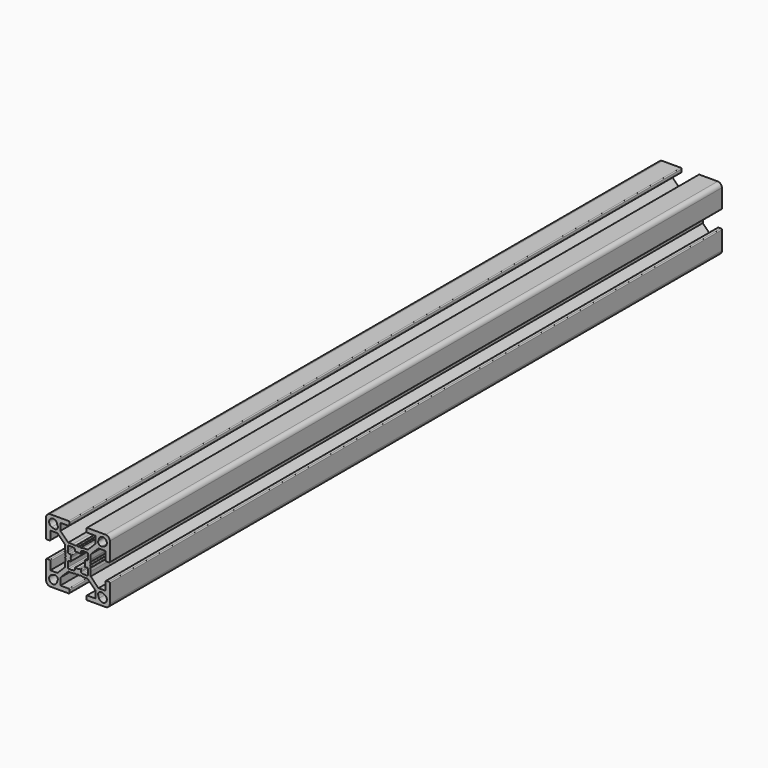
from build123d import *

# Parameters (mm, degrees)
F1_DEPTH = 360


# Not quite as in the source:
# - ends of sketch curves that miss each other by under 0.0002 mm in the source are joined


with BuildPart() as f1:
    # F0 (on Front) → F1 (new body)
    with BuildSketch(Plane.XZ):
        with BuildLine():
            ThreePointArc((21.683673, 22.959406), (21.8008302875, 23.2422487125), (22.083673, 23.359406))
            Line((22.083673, 23.359406), (23.829607, 23.359406))
            ThreePointArc((23.829607, 23.359406), (23.8679454853, 23.3575644616), (23.9059309617, 23.3520568027))
            Line((23.9059309617, 23.3520568027), (24.659993, 23.205482))
            ThreePointArc((24.659993, 23.205482), (24.8923196389, 23.067262524), (24.98367, 22.812831))
            Line((24.98367, 22.812831), (24.98367, 22.196712))
            ThreePointArc((24.98367, 22.196712), (25.1452540389, 21.8755300741), (25.4994591475, 21.8138375123))
            ThreePointArc((25.4994591475, 21.8138375123), (25.9862111121, 21.9228171635), (26.48367, 21.959406))
            Line((26.48367, 21.959406), (26.48367, 24.259406))
            Line((26.48367, 24.259406), (26.080079, 24.492418))
            ThreePointArc((26.080079, 24.492418), (25.830079, 24.559406), (25.5800791291, 24.4924187764))
            Line((25.5800791291, 24.4924187764), (25.264783, 24.310382))
            Line((25.264783, 24.310382), (23.98367, 24.559406))
            Line((23.98367, 24.559406), (21.897875, 24.559406))
            Line((21.897875, 24.559406), (18.23367, 28.223612))
            Line((18.23367, 28.223612), (18.23367, 31.559402))
            Line((18.23367, 31.559402), (22.083673, 31.559402))
            ThreePointArc((22.083673, 31.559402), (22.3665157125, 31.6765592875), (22.483673, 31.959402))
            Line((22.483673, 31.959402), (22.483673, 33.159402))
            ThreePointArc((22.483673, 33.159402), (22.3665157125, 33.4422447125), (22.083673, 33.559402))
            Line((22.083673, 33.559402), (13.483674, 33.559402))
            ThreePointArc((13.483674, 33.559402), (12.0694604376, 32.9736155624), (11.483674, 31.559402))
            Line((11.483674, 31.559402), (11.483674, 22.959403))
            ThreePointArc((11.483674, 22.959403), (11.6008312875, 22.6765602875), (11.883674, 22.559403))
            Line((11.883674, 22.559403), (13.083674, 22.559403))
            ThreePointArc((13.083674, 22.559403), (13.3665167125, 22.6765602875), (13.483674, 22.959403))
            Line((13.483674, 22.959403), (13.483674, 26.809406))
            Line((13.483674, 26.809406), (16.819447, 26.809406))
            Line((16.819447, 26.809406), (20.48367, 23.145184))
            Line((20.48367, 23.145184), (20.48367, 21.059406))
            Line((20.48367, 21.059406), (20.732693, 19.778291))
            Line((20.732693, 19.778291), (20.550657, 19.462994))
            ThreePointArc((20.550657, 19.462994), (20.48367, 19.212994), (20.5506572236, 18.9629941291))
            Line((20.5506572236, 18.9629941291), (20.78367, 18.559405))
            Line((20.78367, 18.559405), (23.08367, 18.559406))
            ThreePointArc((23.08367, 18.559406), (23.1202587453, 19.0568642713), (23.2292374892, 19.543615852))
            ThreePointArc((23.2292374892, 19.543615852), (23.1675451248, 19.897821693), (22.846363, 20.059406))
            Line((22.846363, 20.059406), (22.230245, 20.059406))
            ThreePointArc((22.230245, 20.059406), (21.9758138548, 20.1507560489), (21.8375941973, 20.3830820383))
            Line((21.8375941973, 20.3830820383), (21.691022, 21.137129))
            ThreePointArc((21.691022, 21.137129), (21.6855145384, 21.1751145147), (21.683673, 21.213453))
            Line((21.683673, 21.213453), (21.683673, 22.959406))
        make_face()
        with BuildLine():
            ThreePointArc((14.1338310917, 28.473990252), (13.440167448, 31.6029092165), (16.5690860694, 30.9092440253))
            Line((16.5690860694, 30.9092440253), (16.935818, 29.901655))
            ThreePointArc((16.935818, 29.901655), (16.610197705, 28.4328777176), (15.1414197615, 28.1072573447))
            Line((15.1414197615, 28.1072573447), (14.1338310917, 28.473990252))
        make_face(mode=Mode.SUBTRACT)
        with BuildLine():
            Line((26.48367, 24.259406), (26.48367, 21.959406))
            ThreePointArc((26.48367, 21.959406), (26.9811284145, 21.9228172335), (27.4678801291, 21.813838427))
            ThreePointArc((27.4678801291, 21.813838427), (27.8220855768, 21.8755297889), (27.98367, 22.196712))
            Line((27.98367, 22.196712), (27.98367, 22.812831))
            ThreePointArc((27.98367, 22.812831), (28.0750200489, 23.0672621452), (28.3073460383, 23.2054818027))
            Line((28.3073460383, 23.2054818027), (29.061393, 23.352053))
            ThreePointArc((29.061393, 23.352053), (29.0993785147, 23.3575614616), (29.137717, 23.359403))
            Line((29.137717, 23.359403), (30.88367, 23.359403))
            ThreePointArc((30.88367, 23.359403), (31.1665127125, 23.2422457125), (31.28367, 22.959403))
            Line((31.28367, 22.959403), (31.28367, 21.213468))
            ThreePointArc((31.28367, 21.213468), (31.2818285086, 21.1751300032), (31.27632099, 21.1371450019))
            Line((31.27632099, 21.1371450019), (31.129746, 20.383082))
            ThreePointArc((31.129746, 20.383082), (30.9915261452, 20.1507560489), (30.737095, 20.059406))
            Line((30.737095, 20.059406), (30.120976, 20.059406))
            ThreePointArc((30.120976, 20.059406), (29.7997937889, 19.8978215768), (29.7381017894, 19.5436159363))
            ThreePointArc((29.7381017894, 19.5436159363), (29.8470812335, 19.0568644145), (29.88367, 18.559406))
            Line((29.88367, 18.559406), (32.18367, 18.559406))
            Line((32.18367, 18.559406), (32.416682, 18.962996))
            ThreePointArc((32.416682, 18.962996), (32.48367, 19.212996), (32.4166825264, 19.4629963039))
            Line((32.4166825264, 19.4629963039), (32.234646, 19.778292))
            Line((32.234646, 19.778292), (32.48367, 21.059406))
            Line((32.48367, 21.059406), (32.48367, 23.1452))
            Line((32.48367, 23.1452), (36.147876, 26.809406))
            Line((36.147876, 26.809406), (39.483666, 26.809406))
            Line((39.483666, 26.809406), (39.483666, 22.959403))
            ThreePointArc((39.483666, 22.959403), (39.6008232875, 22.6765602875), (39.883666, 22.559403))
            Line((39.883666, 22.559403), (41.083666, 22.559403))
            ThreePointArc((41.083666, 22.559403), (41.3665087125, 22.6765602875), (41.483666, 22.959403))
            Line((41.483666, 22.959403), (41.483666, 31.559402))
            ThreePointArc((41.483666, 31.559402), (40.8978795624, 32.9736155624), (39.483666, 33.559402))
            Line((39.483666, 33.559402), (30.883667, 33.559402))
            ThreePointArc((30.883667, 33.559402), (30.6008242875, 33.4422447125), (30.483667, 33.159402))
            Line((30.483667, 33.159402), (30.483667, 31.959402))
            ThreePointArc((30.483667, 31.959402), (30.6008242875, 31.6765592875), (30.883667, 31.559402))
            Line((30.883667, 31.559402), (34.73367, 31.559402))
            Line((34.73367, 31.559402), (34.73367, 28.223628))
            Line((34.73367, 28.223628), (31.069448, 24.559406))
            Line((31.069448, 24.559406), (28.98367, 24.559406))
            Line((28.98367, 24.559406), (27.702555, 24.310382))
            Line((27.702555, 24.310382), (27.387259, 24.492418))
            ThreePointArc((27.387259, 24.492418), (27.137259, 24.559406), (26.8872591291, 24.4924187764))
            Line((26.8872591291, 24.4924187764), (26.48367, 24.259406))
        make_face()
        with BuildLine():
            ThreePointArc((36.3982539306, 30.9092440253), (39.5271728843, 31.6029088843), (38.8335080253, 28.4739899306))
            Line((38.8335080253, 28.4739899306), (37.825919, 28.107257))
            ThreePointArc((37.825919, 28.107257), (36.3571411741, 28.4328778386), (36.0315216661, 29.9016561215))
            Line((36.0315216661, 29.9016561215), (36.3982539306, 30.9092440253))
        make_face(mode=Mode.SUBTRACT)
        with BuildLine():
            ThreePointArc((23.2292377663, 17.5751952317), (23.1202588153, 18.0619472552), (23.08367, 18.559406))
            Line((23.08367, 18.559406), (20.78367, 18.559406))
            Line((20.78367, 18.559406), (20.550657, 18.155815))
            ThreePointArc((20.550657, 18.155815), (20.48367, 17.905815), (20.5506572236, 17.6558151291))
            Line((20.5506572236, 17.6558151291), (20.732693, 17.340519))
            Line((20.732693, 17.340519), (20.48367, 16.059406))
            Line((20.48367, 16.059406), (20.48367, 13.973611))
            Line((20.48367, 13.973611), (16.819464, 10.309406))
            Line((16.819464, 10.309406), (13.483674, 10.309406))
            Line((13.483674, 10.309406), (13.483674, 14.159409))
            ThreePointArc((13.483674, 14.159409), (13.3665167125, 14.4422517125), (13.083674, 14.559409))
            Line((13.083674, 14.559409), (11.883674, 14.559409))
            ThreePointArc((11.883674, 14.559409), (11.6008312875, 14.4422517125), (11.483674, 14.159409))
            Line((11.483674, 14.159409), (11.483674, 5.55941))
            ThreePointArc((11.483674, 5.55941), (12.0694604376, 4.1451964376), (13.483674, 3.55941))
            Line((13.483674, 3.55941), (22.083673, 3.55941))
            ThreePointArc((22.083673, 3.55941), (22.3665157125, 3.6765672875), (22.483673, 3.95941))
            Line((22.483673, 3.95941), (22.483673, 5.15941))
            ThreePointArc((22.483673, 5.15941), (22.3665157125, 5.4422527125), (22.083673, 5.55941))
            Line((22.083673, 5.55941), (18.23367, 5.55941))
            Line((18.23367, 5.55941), (18.23367, 8.895183))
            Line((18.23367, 8.895183), (21.897891, 12.559406))
            Line((21.897891, 12.559406), (23.98367, 12.559406))
            Line((23.98367, 12.559406), (25.264785, 12.808429))
            Line((25.264785, 12.808429), (25.580081, 12.626393))
            ThreePointArc((25.580081, 12.626393), (25.830081, 12.559406), (26.0800808709, 12.6263932236))
            Line((26.0800808709, 12.6263932236), (26.483671, 12.859406))
            Line((26.483671, 12.859406), (26.48367, 15.159406))
            ThreePointArc((26.48367, 15.159406), (25.9862111121, 15.1959948365), (25.4994589547, 15.3049738501))
            ThreePointArc((25.4994589547, 15.3049738501), (25.1452540389, 15.2432809259), (24.98367, 14.922099))
            Line((24.98367, 14.922099), (24.98367, 14.305981))
            ThreePointArc((24.98367, 14.305981), (24.8923196389, 14.051549476), (24.6599929981, 13.91333001))
            Line((24.6599929981, 13.91333001), (23.905946, 13.766758))
            ThreePointArc((23.905946, 13.766758), (23.8679609968, 13.7612504914), (23.829623, 13.759409))
            Line((23.829623, 13.759409), (22.08367, 13.759409))
            ThreePointArc((22.08367, 13.759409), (21.8008272875, 13.8765662875), (21.68367, 14.159409))
            Line((21.68367, 14.159409), (21.68367, 15.905343))
            ThreePointArc((21.68367, 15.905343), (21.6855115384, 15.9436814853), (21.6910191973, 15.9816669617))
            Line((21.6910191973, 15.9816669617), (21.837594, 16.735729))
            ThreePointArc((21.837594, 16.735729), (21.975813476, 16.9680556389), (22.230245, 17.059406))
            Line((22.230245, 17.059406), (22.846363, 17.059406))
            ThreePointArc((22.846363, 17.059406), (23.1675448396, 17.2209899227), (23.2292377663, 17.5751952317))
        make_face()
        with BuildLine():
            ThreePointArc((16.5690860694, 6.2095679747), (13.440167448, 5.5159027835), (14.1338310917, 8.644821748))
            Line((14.1338310917, 8.644821748), (15.14142, 9.011554))
            ThreePointArc((15.14142, 9.011554), (16.6101974937, 8.6859334937), (16.9358177723, 7.2171560829))
            Line((16.9358177723, 7.2171560829), (16.5690860694, 6.2095679747))
        make_face(mode=Mode.SUBTRACT)
        with BuildLine():
            ThreePointArc((27.4678801291, 15.304973573), (26.9811284145, 15.1959947665), (26.48367, 15.159406))
            Line((26.48367, 15.159406), (26.48367, 12.859406))
            Line((26.48367, 12.859406), (26.887261, 12.626393))
            ThreePointArc((26.887261, 12.626393), (27.137261, 12.559406), (27.3872608709, 12.6263932236))
            Line((27.3872608709, 12.6263932236), (27.702556, 12.808429))
            Line((27.702556, 12.808429), (28.98367, 12.559406))
            Line((28.98367, 12.559406), (31.069464, 12.559406))
            Line((31.069464, 12.559406), (34.73367, 8.8952))
            Line((34.73367, 8.8952), (34.73367, 5.55941))
            Line((34.73367, 5.55941), (30.883667, 5.55941))
            ThreePointArc((30.883667, 5.55941), (30.6008242875, 5.4422527125), (30.483667, 5.15941))
            Line((30.483667, 5.15941), (30.483667, 3.95941))
            ThreePointArc((30.483667, 3.95941), (30.6008242875, 3.6765672875), (30.883667, 3.55941))
            Line((30.883667, 3.55941), (39.483666, 3.55941))
            ThreePointArc((39.483666, 3.55941), (40.8978795624, 4.1451964376), (41.483666, 5.55941))
            Line((41.483666, 5.55941), (41.483666, 14.159409))
            ThreePointArc((41.483666, 14.159409), (41.3665087125, 14.4422517125), (41.083666, 14.559409))
            Line((41.083666, 14.559409), (39.883666, 14.559409))
            ThreePointArc((39.883666, 14.559409), (39.6008232875, 14.4422517125), (39.483666, 14.159409))
            Line((39.483666, 14.159409), (39.483666, 10.309406))
            Line((39.483666, 10.309406), (36.147892, 10.309406))
            Line((36.147892, 10.309406), (32.48367, 13.973627))
            Line((32.48367, 13.973627), (32.48367, 16.059406))
            Line((32.48367, 16.059406), (32.234646, 17.340521))
            Line((32.234646, 17.340521), (32.416682, 17.655817))
            ThreePointArc((32.416682, 17.655817), (32.48367, 17.905817), (32.4166825264, 18.1558173039))
            Line((32.4166825264, 18.1558173039), (32.18367, 18.559407))
            Line((32.18367, 18.559407), (29.88367, 18.559406))
            ThreePointArc((29.88367, 18.559406), (29.8470811635, 18.0619471121), (29.7381021499, 17.5751949547))
            ThreePointArc((29.7381021499, 17.5751949547), (29.7997940741, 17.2209900389), (30.120976, 17.059406))
            Line((30.120976, 17.059406), (30.737095, 17.059406))
            ThreePointArc((30.737095, 17.059406), (30.991526524, 16.9680556389), (31.12974599, 16.7357289981))
            Line((31.12974599, 16.7357289981), (31.276318, 15.981682))
            ThreePointArc((31.276318, 15.981682), (31.2818255086, 15.9436969968), (31.283667, 15.905359))
            Line((31.283667, 15.905359), (31.283667, 14.159406))
            ThreePointArc((31.283667, 14.159406), (31.1665097125, 13.8765632875), (30.883667, 13.759406))
            Line((30.883667, 13.759406), (29.137732, 13.759406))
            ThreePointArc((29.137732, 13.759406), (29.0993940032, 13.7612474914), (29.0614090019, 13.76675501))
            Line((29.0614090019, 13.76675501), (28.307346, 13.91333))
            ThreePointArc((28.307346, 13.91333), (28.0750200489, 14.0515498548), (27.98367, 14.305981))
            Line((27.98367, 14.305981), (27.98367, 14.922099))
            ThreePointArc((27.98367, 14.922099), (27.8220855768, 15.2432812111), (27.4678801291, 15.304973573))
        make_face()
        with BuildLine():
            ThreePointArc((38.8335080253, 8.6448220694), (39.5271728843, 5.5159031157), (36.3982539306, 6.2095679747))
            Line((36.3982539306, 6.2095679747), (36.031521, 7.217156))
            ThreePointArc((36.031521, 7.217156), (36.3571413854, 8.6859333727), (37.8259189171, 9.0115537723))
            Line((37.8259189171, 9.0115537723), (38.8335080253, 8.6448220694))
        make_face(mode=Mode.SUBTRACT)
    extrude(amount=F1_DEPTH)


solid = f1.part
